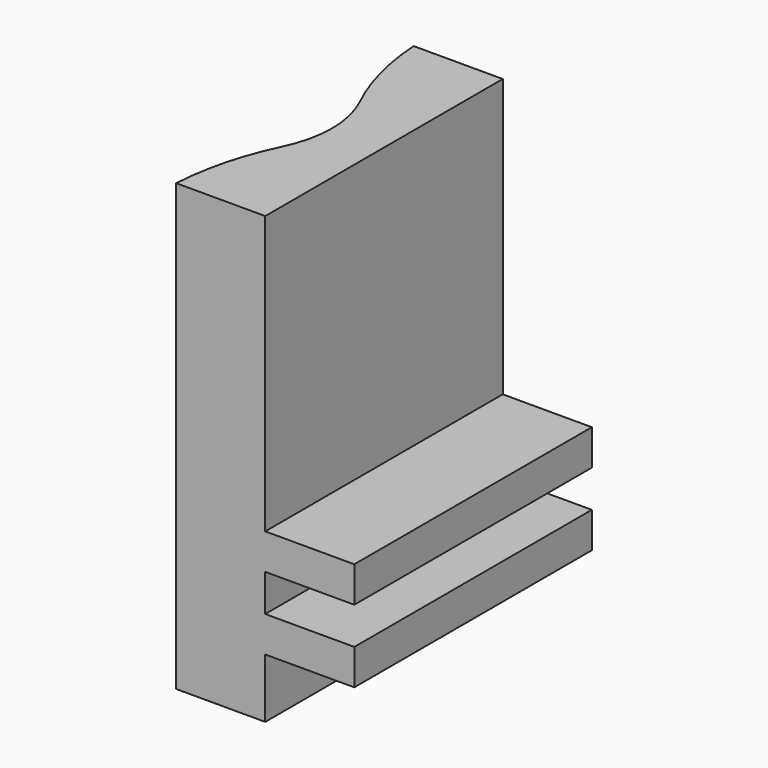
from build123d import *

# Parameters (mm, degrees)
F1_DEPTH    = 25.4
F2_T1_DEPTH = 53.4024208572
F3_DEPTH    = 10.16
F4_DEPTH    = 2.54
F5_W        = 25.4
F5_H        = 3.048
F6_DEPTH    = 7.62
F8_DEPTH    = 5.08


# Not quite as in the source:
# - a fillet or chamfer that OpenCascade refuses, or shapes differently, is made with other operations: its cross-section is extruded or revolved along the edge and cut away or added


with BuildPart() as f1:
    # F0 (on Top) → F1 (new body)
    with BuildSketch(Plane.XY):
        with BuildLine():
            Line((-3.81, -12.7), (3.81, -12.7))
            Line((3.81, -12.7), (3.81, 12.7))
            Line((3.81, 12.7), (-3.81, 12.7))
            Line((-3.81, 12.7), (-3.81, 7.0995158286))
            ThreePointArc((-3.81, 7.0995158286), (-1.4649043996, 3.8885649667), (-0.635, 0))
            ThreePointArc((-0.635, 0), (-1.4649043996, -3.8885649667), (-3.81, -7.0995158286))
            Line((-3.81, -7.0995158286), (-3.81, -12.7))
        make_face()
    extrude(amount=F1_DEPTH)

    # F2: fillet of radius 22.86 on 2 edges, made by hand

    # F2_s2 → F2_t1 (cut)
    with BuildSketch(Plane.XY.offset(-14.0012104286)):
        with BuildLine():
            ThreePointArc((-3.81, 12.7), (-3.1136000163, 8.3102394823), (-1.5809070588, 4.1382108824))
            ThreePointArc((-1.5809070588, 4.1382108824), (-2.5500206467, 5.7283365162), (-3.81, 7.0995158286))
            Line((-3.81, 7.0995158286), (-3.81, 12.7))
        make_face()
        with BuildLine():
            ThreePointArc((-3.81, -12.7), (-3.1136000163, -8.3102394823), (-1.5809070588, -4.1382108824))
            ThreePointArc((-1.5809070588, -4.1382108824), (-2.5500206467, -5.7283365162), (-3.81, -7.0995158286))
            Line((-3.81, -7.0995158286), (-3.81, -12.7))
        make_face()
    extrude(amount=F2_T1_DEPTH, mode=Mode.SUBTRACT)

    # F3 (add): a face of the model
    f3_faces = [f1.faces().sort_by_distance(p)[0] for p in [
        (0.6414875327, 0, 25.4),
    ]]
    extrude(f3_faces, amount=F3_DEPTH)

    # F4 (add): a face of the model
    f4_faces = [f1.faces().sort_by_distance(p)[0] for p in [
        (0.6414875327, 0, 35.56),
    ]]
    extrude(f4_faces, amount=F4_DEPTH)

    # F5 (on face) → F6 (join)
    with BuildSketch(Plane.YZ.offset(3.81)):
        with Locations((0, 12.827)):
            Rectangle(F5_W, F5_H)
        with Locations((0, 6.604)):
            Rectangle(F5_W, F5_H)
    extrude(amount=F6_DEPTH)

    # F7 (on face) → F8 (join)
    with BuildSketch(Plane.XY.offset(8.128)):
        with BuildLine():
            ThreePointArc((3.81, -4.572), (6.427457728, -1.435728864), (7.366, 2.54))
            ThreePointArc((7.366, 2.54), (6.427457728, 6.515728864), (3.81, 9.652))
            Line((3.81, 9.652), (3.81, -4.572))
        make_face()
    extrude(amount=F8_DEPTH)


solid = f1.part
